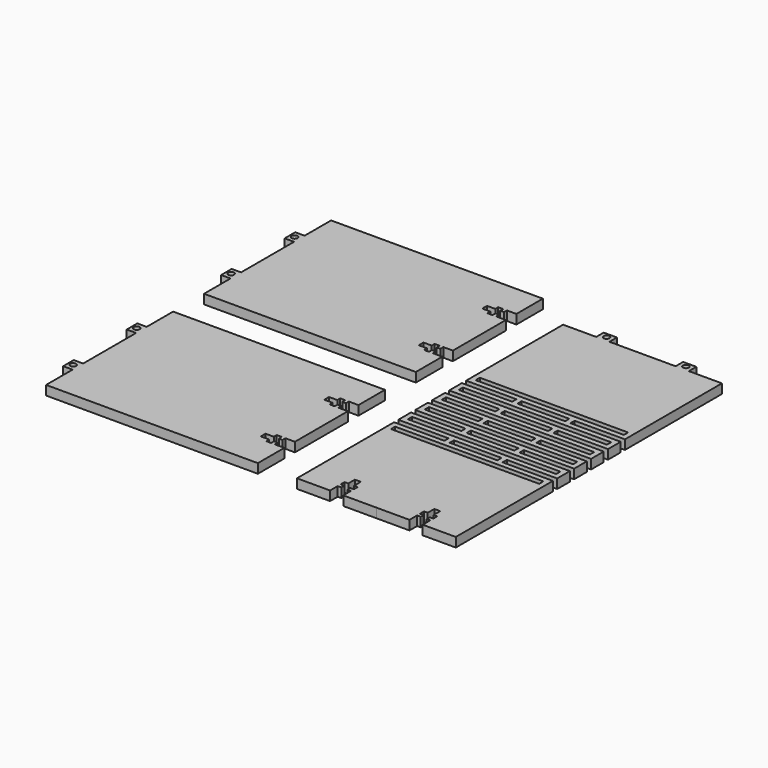
from build123d import *

# Parameters (mm, degrees)
F0_R     = 1.4224
F1_DEPTH = 4.4958
F2_DEPTH = 4.4958


# Not quite as in the source:
# - ends of sketch curves that miss each other by under 0.0002 mm in the source are joined


with BuildPart() as f1:
    # F0 (on Top) → F1 (new body)
    with BuildSketch(Plane.XY):
        Polygon((85.6072632492, 31.7115586693), (69.7322632492, 31.7115586693), (69.7322632492, -21.3744413307), (105.2922632492, -21.3744413307), (105.2922632492, -23.9144413307), (83.7022632492, -23.9144413307), (83.5963865209, -23.9144413307), (69.7322632492, -23.9144413307), (69.7322632492, -26.4544413307), (81.162649971, -26.4544413307), (81.162649971, -28.9944413307), (69.7322632492, -28.9944413307), (69.7322632492, -31.5344413307), (83.7022632712, -31.5344413307), (105.2922632492, -31.5344413307), (105.2922632492, -34.0744413307), (83.7022632492, -34.0744413307), (83.5963865209, -34.0744413307), (69.7322632492, -34.0744413307), (69.7322632492, -36.6144413307), (81.162649971, -36.6144413307), (81.162649971, -39.1544413307), (69.7322632492, -39.1544413307), (69.7322632492, -41.6944413307), (83.7022632712, -41.6944413307), (105.2922632492, -41.6944413307), (105.2922632492, -44.2344413307), (83.7022632492, -44.2344413307), (83.5963865209, -44.2344413307), (69.7322632492, -44.2344413307), (69.7322632492, -46.7744413307), (81.162649971, -46.7744413307), (81.162649971, -49.3144413307), (69.7322632492, -49.3144413307), (69.7322632492, -51.8544413307), (83.7022632712, -51.8544413307), (105.2922632492, -51.8544413307), (105.2922632492, -54.3944413307), (83.7022632492, -54.3944413307), (83.5963865209, -54.3944413307), (69.7322632492, -54.3944413307), (69.7322632492, -56.9344413307), (81.162649971, -56.9344413307), (81.162649971, -59.4744413307), (69.7322632492, -59.4744413307), (69.7322632492, -62.0144413307), (83.7022632712, -62.0144413307), (105.2922632492, -62.0144413307), (105.2922632492, -64.5544413307), (83.7022632492, -64.5544413307), (83.5963865209, -64.5544413307), (69.7322632492, -64.5544413307), (69.7322632492, -67.0944413307), (81.162649971, -67.0944413307), (81.162649971, -69.6344413307), (69.7322632492, -69.6344413307), (69.7322632492, -72.1744413307), (83.7022632712, -72.1744413307), (105.2922632492, -72.1744413307), (105.2922632492, -74.7144413307), (69.7322632492, -74.7144413307), (69.7322632492, -127.8813485955), (85.60218325, -127.8813481331), (85.6022909453, -123.3091983183), (87.3600128259, -123.3091983183), (87.3600128259, -121.5312732244), (85.6075624026, -121.5312732244), (85.6075624026, -119.1500232244), (87.3598632492, -119.1500232244), (87.3598632492, -115.1812732244), (90.2046632492, -115.1812732244), (90.2046632492, -119.1500232244), (91.9572632492, -119.1500232244), (91.9572632492, -121.5312732244), (90.2048128259, -121.5312732244), (90.2048128259, -123.3091983183), (91.9624509471, -123.3091983183), (91.9623432483, -127.8813481331), (107.8322632492, -127.8813481331), (107.8322632492, -69.6344413307), (83.7022632712, -69.6344413307), (83.7022632712, -67.0944413307), (107.8322632492, -67.0944413307), (107.8322632492, -59.4744413307), (83.7022632712, -59.4744413307), (83.7022632712, -56.9344413307), (107.8322632492, -56.9344413307), (107.8322632492, -49.3144413307), (83.7022632712, -49.3144413307), (83.7022632712, -46.7744413307), (107.8322632492, -46.7744413307), (107.8322632492, -39.1544413307), (83.7022632712, -39.1544413307), (83.7022632712, -36.6144413307), (107.8322632492, -36.6144413307), (107.8322632492, -28.9944413307), (83.7022632712, -28.9944413307), (83.7022632712, -26.4544413307), (107.8322632492, -26.4544413307), (107.8322632492, -21.3744413307), (107.8322632492, 31.7115586693), (91.9572632492, 31.7115586693), (91.9572632492, 36.2073586693), (85.6072632492, 36.2073586693), align=None)
        with Locations((88.7822632492, 33.9594586693)):
            Circle(F0_R, mode=Mode.SUBTRACT)
    extrude(amount=F1_DEPTH)

    # F0 (on Top) → F2, piece 2 (join)
    with BuildSketch(Plane.XY):
        Polygon((47.5072632492, 31.7115586693), (31.6322632492, 31.7115586693), (31.6322632492, -21.3744413307), (31.6322632492, -26.4544413307), (55.7622632271, -26.4544413307), (55.7622632271, -28.9944413307), (31.6322632492, -28.9944413307), (31.6322632492, -36.6144413307), (55.7622632271, -36.6144413307), (55.7622632271, -39.1544413307), (31.6322632492, -39.1544413307), (31.6322632492, -46.7744413307), (55.7622632271, -46.7744413307), (55.7622632271, -49.3144413307), (31.6322632492, -49.3144413307), (31.6322632492, -56.9344413307), (55.7622632271, -56.9344413307), (55.7622632271, -59.4744413307), (31.6322632492, -59.4744413307), (31.6322632492, -67.0944413307), (55.7622632271, -67.0944413307), (55.7622632271, -69.6344413307), (31.6322632492, -69.6344413307), (31.6322632492, -127.8813481331), (47.50218325, -127.8813481331), (47.5020755513, -123.3091983183), (49.2597136724, -123.3091983183), (49.2597136724, -121.5312732244), (47.5072632492, -121.5312732244), (47.5072632492, -119.1500232244), (49.2598632492, -119.1500232244), (49.2598632492, -115.1812732244), (52.1046632492, -115.1812732244), (52.1046632492, -119.1500232244), (53.8569640957, -119.1500232244), (53.8569640957, -121.5312732244), (52.1045136724, -121.5312732244), (52.1045136724, -123.3091983183), (53.862235553, -123.3091983183), (53.8623432483, -127.8813481331), (69.7322632492, -127.8813481331), (69.7322632492, -74.7144413307), (55.7622632271, -74.7144413307), (34.1722632492, -74.7144413307), (34.1722632492, -72.1744413307), (55.7622632271, -72.1744413307), (69.7322632492, -72.1744413307), (69.7322632492, -69.6344413307), (58.3018765273, -69.6344413307), (58.3018765273, -67.0944413307), (69.7322632492, -67.0944413307), (69.7322632492, -64.5544413307), (55.8681399775, -64.5544413307), (55.7622632492, -64.5544413307), (34.1722632492, -64.5544413307), (34.1722632492, -62.0144413307), (55.7622632271, -62.0144413307), (69.7322632492, -62.0144413307), (69.7322632492, -59.4744413307), (58.3018765273, -59.4744413307), (58.3018765273, -56.9344413307), (69.7322632492, -56.9344413307), (69.7322632492, -54.3944413307), (55.8681399775, -54.3944413307), (55.7622632492, -54.3944413307), (34.1722632492, -54.3944413307), (34.1722632492, -51.8544413307), (55.7622632271, -51.8544413307), (69.7322632492, -51.8544413307), (69.7322632492, -49.3144413307), (58.3018765273, -49.3144413307), (58.3018765273, -46.7744413307), (69.7322632492, -46.7744413307), (69.7322632492, -44.2344413307), (55.8681399775, -44.2344413307), (55.7622632492, -44.2344413307), (34.1722632492, -44.2344413307), (34.1722632492, -41.6944413307), (55.7622632271, -41.6944413307), (69.7322632492, -41.6944413307), (69.7322632492, -39.1544413307), (58.3018765273, -39.1544413307), (58.3018765273, -36.6144413307), (69.7322632492, -36.6144413307), (69.7322632492, -34.0744413307), (55.8681399775, -34.0744413307), (55.7622632492, -34.0744413307), (34.1722632492, -34.0744413307), (34.1722632492, -31.5344413307), (55.7622632271, -31.5344413307), (69.7322632492, -31.5344413307), (69.7322632492, -28.9944413307), (58.3018765273, -28.9944413307), (58.3018765273, -26.4544413307), (69.7322632492, -26.4544413307), (69.7322632492, -23.9144413307), (55.8681399775, -23.9144413307), (55.7622632492, -23.9144413307), (34.1722632492, -23.9144413307), (34.1722632492, -21.3744413307), (69.7322632492, -21.3744413307), (69.7322632492, 31.7115586693), (53.8572632492, 31.7115586693), (53.8572632492, 36.2073586693), (47.5072632492, 36.2073586693), align=None)
        with Locations((50.6822632492, 33.9594586693)):
            Circle(F0_R, mode=Mode.SUBTRACT)
        Polygon((85.6072632492, 31.7115586693), (69.7322632492, 31.7115586693), (69.7322632492, -21.3744413307), (105.2922632492, -21.3744413307), (105.2922632492, -23.9144413307), (83.7022632492, -23.9144413307), (83.5963865209, -23.9144413307), (69.7322632492, -23.9144413307), (69.7322632492, -26.4544413307), (81.162649971, -26.4544413307), (81.162649971, -28.9944413307), (69.7322632492, -28.9944413307), (69.7322632492, -31.5344413307), (83.7022632712, -31.5344413307), (105.2922632492, -31.5344413307), (105.2922632492, -34.0744413307), (83.7022632492, -34.0744413307), (83.5963865209, -34.0744413307), (69.7322632492, -34.0744413307), (69.7322632492, -36.6144413307), (81.162649971, -36.6144413307), (81.162649971, -39.1544413307), (69.7322632492, -39.1544413307), (69.7322632492, -41.6944413307), (83.7022632712, -41.6944413307), (105.2922632492, -41.6944413307), (105.2922632492, -44.2344413307), (83.7022632492, -44.2344413307), (83.5963865209, -44.2344413307), (69.7322632492, -44.2344413307), (69.7322632492, -46.7744413307), (81.162649971, -46.7744413307), (81.162649971, -49.3144413307), (69.7322632492, -49.3144413307), (69.7322632492, -51.8544413307), (83.7022632712, -51.8544413307), (105.2922632492, -51.8544413307), (105.2922632492, -54.3944413307), (83.7022632492, -54.3944413307), (83.5963865209, -54.3944413307), (69.7322632492, -54.3944413307), (69.7322632492, -56.9344413307), (81.162649971, -56.9344413307), (81.162649971, -59.4744413307), (69.7322632492, -59.4744413307), (69.7322632492, -62.0144413307), (83.7022632712, -62.0144413307), (105.2922632492, -62.0144413307), (105.2922632492, -64.5544413307), (83.7022632492, -64.5544413307), (83.5963865209, -64.5544413307), (69.7322632492, -64.5544413307), (69.7322632492, -67.0944413307), (81.162649971, -67.0944413307), (81.162649971, -69.6344413307), (69.7322632492, -69.6344413307), (69.7322632492, -72.1744413307), (83.7022632712, -72.1744413307), (105.2922632492, -72.1744413307), (105.2922632492, -74.7144413307), (69.7322632492, -74.7144413307), (69.7322632492, -127.8813485955), (85.60218325, -127.8813481331), (85.6022909453, -123.3091983183), (87.3600128259, -123.3091983183), (87.3600128259, -121.5312732244), (85.6075624026, -121.5312732244), (85.6075624026, -119.1500232244), (87.3598632492, -119.1500232244), (87.3598632492, -115.1812732244), (90.2046632492, -115.1812732244), (90.2046632492, -119.1500232244), (91.9572632492, -119.1500232244), (91.9572632492, -121.5312732244), (90.2048128259, -121.5312732244), (90.2048128259, -123.3091983183), (91.9624509471, -123.3091983183), (91.9623432483, -127.8813481331), (107.8322632492, -127.8813481331), (107.8322632492, -69.6344413307), (83.7022632712, -69.6344413307), (83.7022632712, -67.0944413307), (107.8322632492, -67.0944413307), (107.8322632492, -59.4744413307), (83.7022632712, -59.4744413307), (83.7022632712, -56.9344413307), (107.8322632492, -56.9344413307), (107.8322632492, -49.3144413307), (83.7022632712, -49.3144413307), (83.7022632712, -46.7744413307), (107.8322632492, -46.7744413307), (107.8322632492, -39.1544413307), (83.7022632712, -39.1544413307), (83.7022632712, -36.6144413307), (107.8322632492, -36.6144413307), (107.8322632492, -28.9944413307), (83.7022632712, -28.9944413307), (83.7022632712, -26.4544413307), (107.8322632492, -26.4544413307), (107.8322632492, -21.3744413307), (107.8322632492, 31.7115586693), (91.9572632492, 31.7115586693), (91.9572632492, 36.2073586693), (85.6072632492, 36.2073586693), align=None)
        with Locations((88.7822632492, 33.9594586693)):
            Circle(F0_R, mode=Mode.SUBTRACT)
    extrude(amount=F2_DEPTH)


with BuildPart() as f2:
    # F0 (on Top) → F2 (new body)
    with BuildSketch(Plane.XY):
        Polygon((12.5262859201, 43.466242066), (-89.0737140799, 43.466242066), (-89.0737140799, 27.5936352938), (-93.5695140799, 27.5936352938), (-93.5695140799, 21.2436352938), (-89.0737140799, 21.2436352938), (-89.0737140799, -10.5111511618), (-93.5695140799, -10.5111511618), (-93.5695140799, -16.8611511618), (-89.0737140799, -16.8611511618), (-89.0737140799, -32.733757934), (12.5262859201, -32.733757934), (12.5262859201, -16.8638379331), (7.9541361053, -16.8639456319), (7.9541361053, -15.1063075107), (6.1762110114, -15.1063075107), (6.1762110114, -16.858757934), (3.7949610114, -16.858757934), (3.7949610114, -15.106157934), (-0.1737889886, -15.106157934), (-0.1737889886, -12.261357934), (3.7949610114, -12.261357934), (3.7949610114, -10.5090570875), (6.1762110114, -10.5090570875), (6.1762110114, -12.2615075107), (7.9541361053, -12.2615075107), (7.9541361053, -10.5037856301), (12.5262859201, -10.5036779349), (12.5262859201, 21.2361620669), (7.9541361053, 21.2362697622), (7.9541361053, 22.9939916428), (6.1762110114, 22.9939916428), (6.1762110114, 21.2415412195), (3.7949610114, 21.2415412195), (3.7949610114, 22.993842066), (-0.1737889886, 22.993842066), (-0.1737889886, 25.838642066), (3.7949610114, 25.838642066), (3.7949610114, 27.591242066), (6.1762110114, 27.591242066), (6.1762110114, 25.8387916428), (7.9541361053, 25.8387916428), (7.9541361053, 27.5964297639), (12.5262859201, 27.5963220651), align=None)
        with Locations((-91.3216140799, -13.6861511618)):
            Circle(F0_R, mode=Mode.SUBTRACT)
        with Locations((-91.3216140799, 24.4186352938)):
            Circle(F0_R, mode=Mode.SUBTRACT)
    extrude(amount=F2_DEPTH)


with BuildPart() as f2b:
    # F0 (on Top) → F2, piece 3 (new body)
    with BuildSketch(Plane.XY):
        Polygon((7.9541361053, -73.4816533374), (7.9541361053, -71.7239314568), (6.1762110114, -71.7239314568), (6.1762110114, -73.47638188), (3.7949610114, -73.47638188), (3.7949610114, -71.7240810335), (-0.1737889886, -71.7240810335), (-0.1737889886, -68.8792810335), (3.7949610114, -68.8792810335), (3.7949610114, -67.1266810335), (6.1762110114, -67.1266810335), (6.1762110114, -68.8791314568), (7.9541361053, -68.8791314568), (7.9541361053, -67.1214933356), (12.5262859201, -67.1216010344), (12.5262859201, -51.2516810335), (-89.0737140799, -51.2516810335), (-89.0737140799, -67.1242878057), (-93.5695140799, -67.1242878057), (-93.5695140799, -73.4742878057), (-89.0737140799, -73.4742878057), (-89.0737140799, -105.2290742613), (-93.5695140799, -105.2290742613), (-93.5695140799, -111.5790742613), (-89.0737140799, -111.5790742613), (-89.0737140799, -127.4516810335), (12.5262859201, -127.4516810335), (12.5262859201, -111.5817610326), (7.9541361053, -111.5818687314), (7.9541361053, -109.8242306103), (6.1762110114, -109.8242306103), (6.1762110114, -111.5766810335), (3.7949610114, -111.5766810335), (3.7949610114, -109.8240810335), (-0.1737889886, -109.8240810335), (-0.1737889886, -106.9792810335), (3.7949610114, -106.9792810335), (3.7949610114, -105.226980187), (6.1762110114, -105.226980187), (6.1762110114, -106.9794306103), (7.9541361053, -106.9794306103), (7.9541361053, -105.2217087297), (12.5262859201, -105.2216010344), (12.5262859201, -73.4817610326), align=None)
        with Locations((-91.3216140799, -108.4040742613)):
            Circle(F0_R, mode=Mode.SUBTRACT)
        with Locations((-91.3216140799, -70.2992878057)):
            Circle(F0_R, mode=Mode.SUBTRACT)
    extrude(amount=F2_DEPTH)


solid = Compound([f1.part, f2.part, f2b.part])
